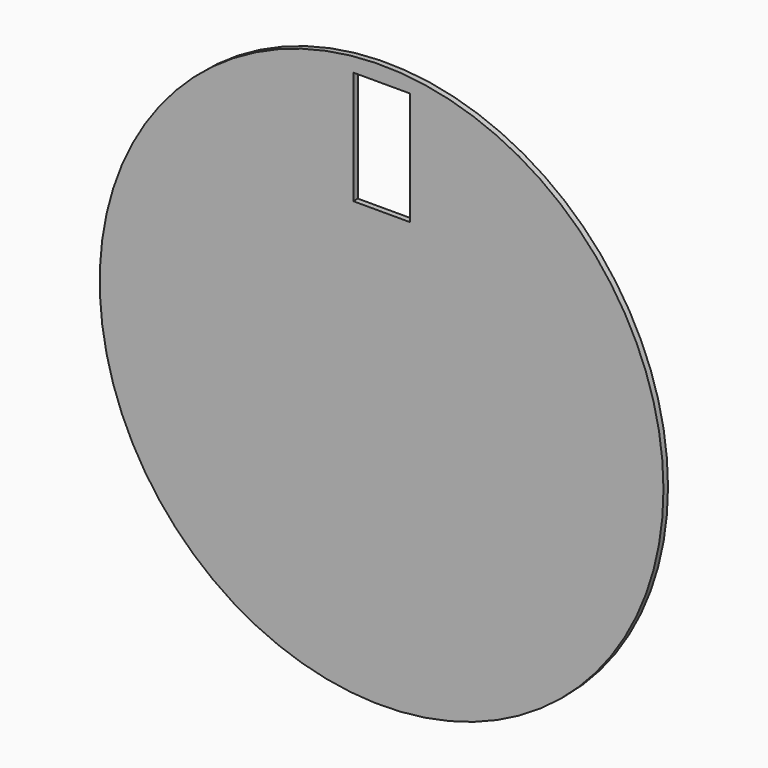
from build123d import *

# Parameters (mm, degrees)
F2_R     = 24.892
F5_DEPTH = 0.5
F1_W     = 5
F1_H     = 10
F6_DEPTH = 2.6162


# Not quite as in the source:
# - the program builds the solid bodies; features that only make, move or delete a surface that nothing else refers to are left out


with BuildPart() as f5:
    # F2 (on Front) → F5 (new body)
    with BuildSketch(Plane.XZ):
        Circle(F2_R)
    extrude(amount=F5_DEPTH)

    # F1 (on Front) → F6 (cut)
    with BuildSketch(Plane.XZ):
        with Locations((0, 18.4979066253)):
            Rectangle(F1_W, F1_H)
    extrude(amount=F6_DEPTH, mode=Mode.SUBTRACT)


solid = f5.part
